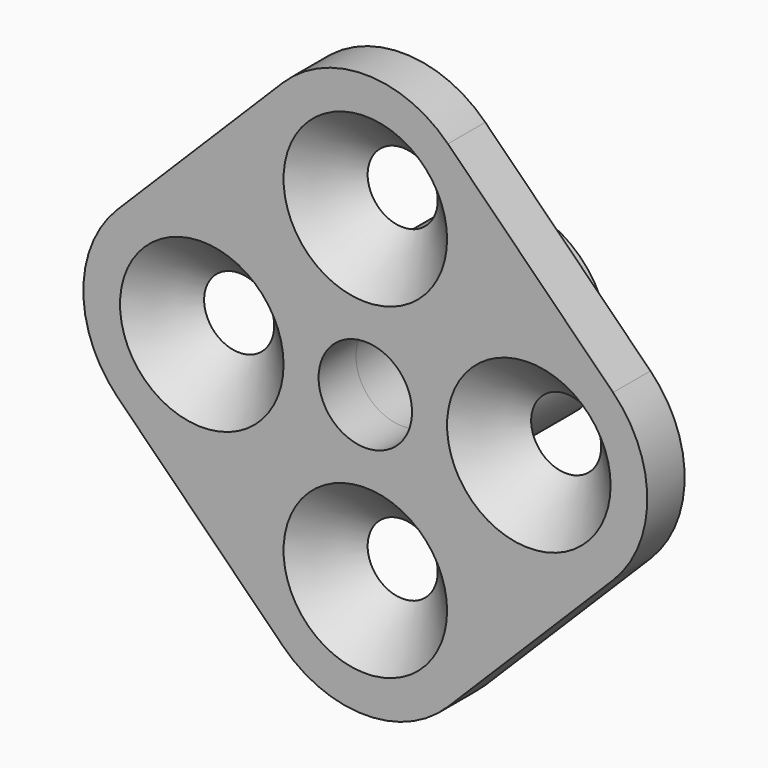
from build123d import *

# Parameters (mm, degrees)
F0_R     = 1.5
F0_R_2   = 2
F1_DEPTH = 2
F2_SIZE  = 1.99999
F3_R     = 4
F3_R_2   = 2
F4_DEPTH = 6


# Not quite as in the source:
# - a fillet or chamfer is up to 0.001 mm smaller than in the source, because OpenCascade refuses the exact size


with BuildPart() as f1:
    # F0 (on Front) → F1 (new body)
    with BuildSketch(Plane.XZ):
        with BuildLine():
            Line((-10.6066017178, -3.5355339059), (-3.5355339059, -10.6066017178))
            ThreePointArc((-3.5355339059, -10.6066017178), (0, -12.0710678119), (3.5355339059, -10.6066017178))
            Line((3.5355339059, -10.6066017178), (10.6066017178, -3.5355339059))
            ThreePointArc((10.6066017178, -3.5355339059), (12.0710678119, 0), (10.6066017178, 3.5355339059))
            Line((10.6066017178, 3.5355339059), (3.5355339059, 10.6066017178))
            ThreePointArc((3.5355339059, 10.6066017178), (0, 12.0710678119), (-3.5355339059, 10.6066017178))
            Line((-3.5355339059, 10.6066017178), (-10.6066017178, 3.5355339059))
            ThreePointArc((-10.6066017178, 3.5355339059), (-12.0710678119, 0), (-10.6066017178, -3.5355339059))
        make_face()
        with Locations((-7, 0)):
            Circle(F0_R, mode=Mode.SUBTRACT)
        with Locations((0, -7)):
            Circle(F0_R, mode=Mode.SUBTRACT)
        Circle(F0_R_2, mode=Mode.SUBTRACT)
        with Locations((7, 0)):
            Circle(F0_R, mode=Mode.SUBTRACT)
        with Locations((0, 7)):
            Circle(F0_R, mode=Mode.SUBTRACT)
    extrude(amount=F1_DEPTH)

    # F2 (size 2 in the source; OpenCascade refuses exactly that, so slightly less here)
    f2_edges = [f1.edges().sort_by_distance(p)[0] for p in [
        (5.5, -2, 0),
        (-1.5, -2, -7),
        (-8.5, -2, 0),
        (-1.5, -2, 7),
    ]]
    chamfer(f2_edges, length=F2_SIZE)

    # F3 (on face) → F4 (join)
    with BuildSketch(Plane(origin=(0, 0, 0), x_dir=(-1, 0, 0), z_dir=(0, 1, 0))):
        Circle(F3_R)
        Circle(F3_R_2, mode=Mode.SUBTRACT)
    extrude(amount=F4_DEPTH)


solid = f1.part
